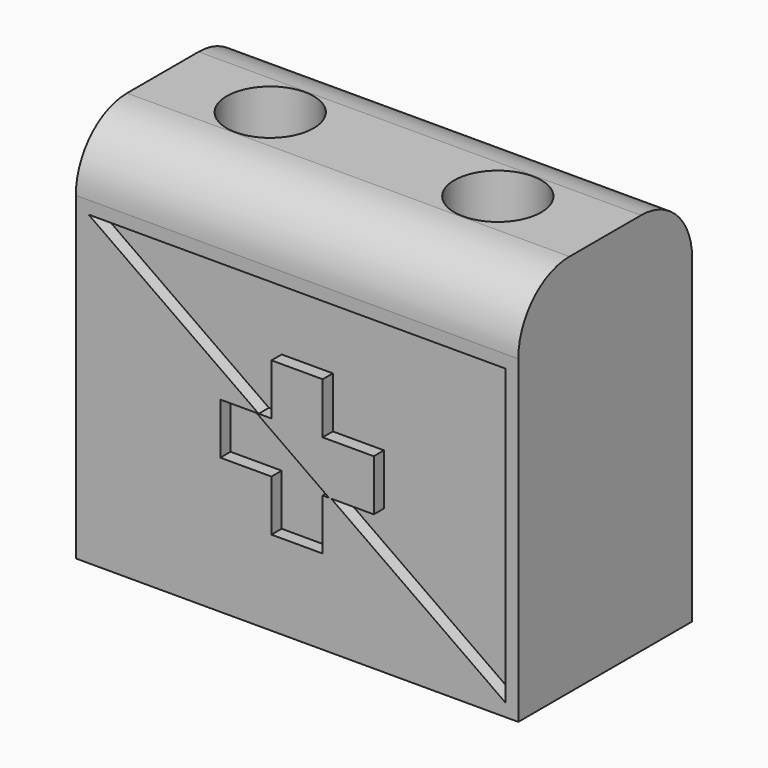
from build123d import *

# Parameters (mm, degrees)
F0_W     = 87.884
F0_H     = 76.2
F1_DEPTH = 43.18
F2_R     = 12.7
F4_DEPTH = 2.54
F5_DEPTH = 2.54
F7_DEPTH = 2.54
F8_R     = 8.636
F9_DEPTH = 76.201


# Not quite as in the source:
# - ends of sketch curves that miss each other by under 0.0002 mm in the source are joined


with BuildPart() as f1:
    # F0 (on Front) → F1 (new body)
    with BuildSketch(Plane.XZ):
        with Locations((43.942, 38.1)):
            Rectangle(F0_W, F0_H)
    extrude(amount=F1_DEPTH)

    # F2
    f2_edges = [f1.edges().sort_by_distance(p)[0] for p in [
        (43.942, -43.18, 76.2),
        (43.942, 0, 76.2),
    ]]
    fillet(f2_edges, radius=F2_R)

    # F3 (on face) → F4 (cut)
    with BuildSketch(Plane.XZ.offset(43.18)):
        Polygon((38.862, 47.2823401565), (43.942, 47.2823401565), (49.022, 47.2823401565), (49.022, 37.1223401565), (59.182, 37.1223401565), (59.182, 26.9623401565), (50.7279873173, 26.9623401565), (85.3440016508, 2.5399983492), (85.3440016508, 60.9600016508), (2.5399983492, 60.9600016508), (36.3272919048, 37.1223401565), (38.862, 37.1223401565), align=None)
    extrude(amount=-F4_DEPTH, mode=Mode.SUBTRACT)

    # F3 (on face) → F5 (cut)
    with BuildSketch(Plane.XZ.offset(43.18)):
        Polygon((50.2873871384, 26.9623401565), (35.8866917258, 37.1223401565), (28.702, 37.1223401565), (28.702, 26.9623401565), (38.862, 26.9623401565), (38.862, 16.8023401565), (43.942, 16.8023401565), (49.022, 16.8023401565), (49.022, 26.9623401565), align=None)
    extrude(amount=-F5_DEPTH, mode=Mode.SUBTRACT)

    # F6 (on face) → F7 (cut)
    with BuildSketch(Plane(origin=(0, 0, 0), x_dir=(-1, 0, 0), z_dir=(0, 1, 0))):
        Polygon((-48.0027233214, 47.2823394346), (-42.9227233214, 47.2823394346), (-37.8427233214, 47.2823394346), (-37.8427233214, 37.1223394346), (-27.6827233214, 37.1223394346), (-27.6827233214, 26.9623394346), (-37.1560138865, 26.9623391642), (-2.54, 2.5399966984), (-2.54, 60.96), (-85.344, 60.96), (-51.5567091082, 37.1223394346), (-48.0027233214, 37.1223394346), align=None)
        Polygon((-37.5966140538, 26.9623391642), (-51.9973092754, 37.1223394346), (-58.1627233214, 37.1223394346), (-58.1627233214, 26.9623394346), (-48.0027233214, 26.9623394346), (-48.0027233214, 16.8023394346), (-42.9227233214, 16.8023394346), (-37.8427233214, 16.8023394346), (-37.8427233214, 26.9623394346), align=None)
    extrude(amount=-F7_DEPTH, mode=Mode.SUBTRACT)

    # F8 (on face) → F9 (cut, through all)
    with BuildSketch(Plane.XY.offset(76.2)):
        with Locations((21.336, -21.59)):
            Circle(F8_R)
        with Locations((66.548, -21.59)):
            Circle(F8_R)
    extrude(amount=-F9_DEPTH, mode=Mode.SUBTRACT)


solid = f1.part
